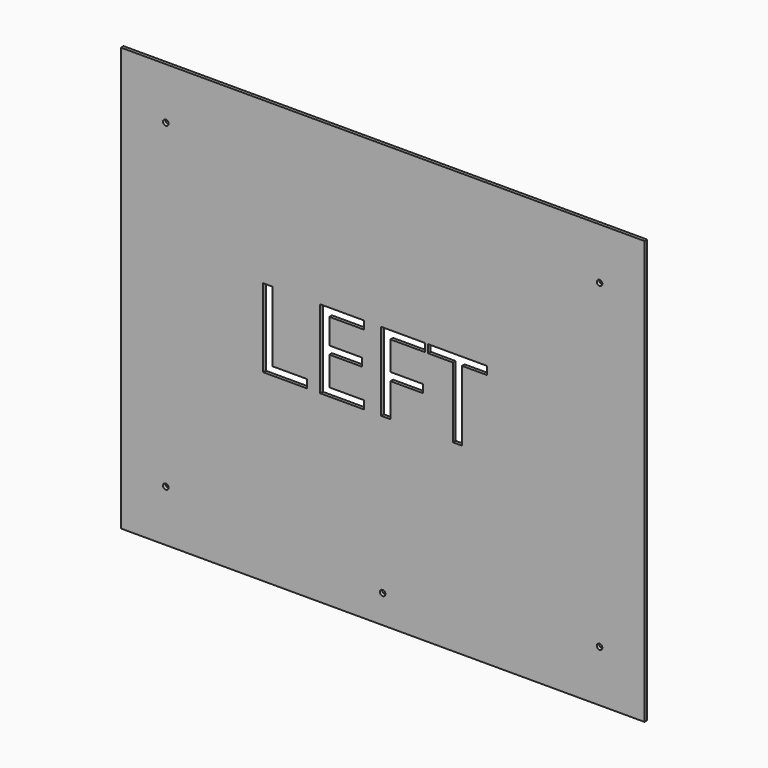
from build123d import *

# Parameters (mm, degrees)
F0_W         = 508.25
F0_H         = 411
F1_DEPTH     = 3.175
F2_TEXT_SIZE = 106.5619574446
F3_DEPTH     = 25
F4_R         = 2.7
F5_DEPTH     = 25


# Not quite as in the source:
# - Text() gives the source's letters only with a copy of the font that has no kerning and outlines rounded to 1/6400 em; it was checked with that copy


with BuildPart() as f1:
    # F0 (on Front) → F1 (new body)
    with BuildSketch(Plane.XZ):
        Rectangle(F0_W, F0_H)
    extrude(amount=F1_DEPTH)

    # F2 (on face) → F3 (cut)
    with BuildSketch(Plane.XZ.offset(3.175)):
        with Locations((-126.433506608, -27.015702799)):
            Text('LEFT', F2_TEXT_SIZE, font='Open Sans', text_align=(TextAlign.LEFT, TextAlign.BOTTOM))
    extrude(amount=-F3_DEPTH, mode=Mode.SUBTRACT)

    # F4 (on face) → F5 (cut)
    with BuildSketch(Plane.XZ.offset(3.175)):
        with Locations((-210.525, 155.5)):
            Circle(F4_R)
        with Locations((-210.525, -155.5)):
            Circle(F4_R)
        with Locations((210.525, 155.5)):
            Circle(F4_R)
        with Locations((210.525, -155.5)):
            Circle(F4_R)
        with Locations((-0.025, -178)):
            Circle(F4_R)
    extrude(amount=-F5_DEPTH, mode=Mode.SUBTRACT)


solid = f1.part
